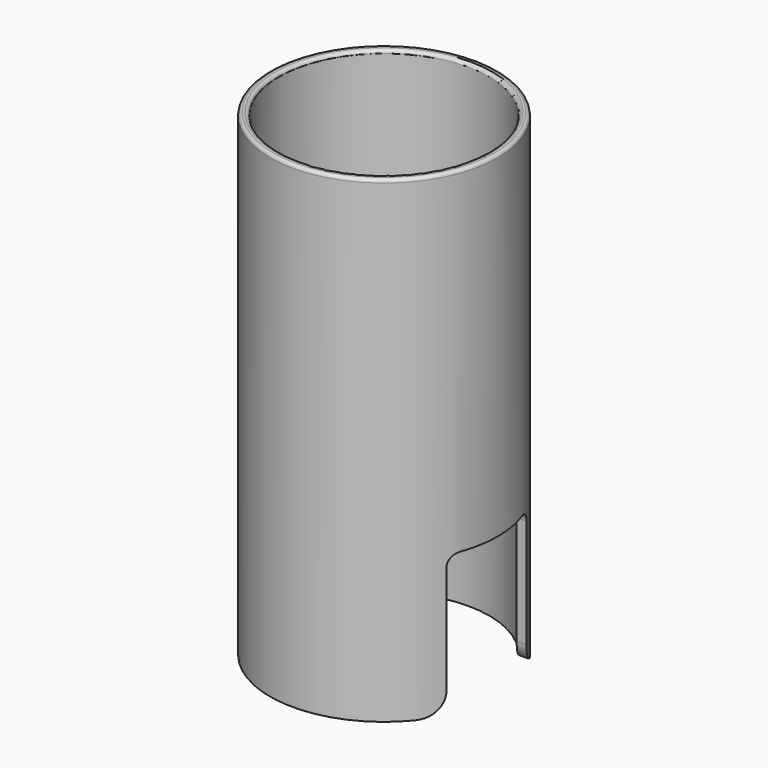
from build123d import *

# Parameters (mm, degrees)
F0_R        = 10.5
F0_R_2      = 9.7
F1_DEPTH    = 44
F3_DEPTH    = 20.75
F4_T1_DEPTH = 10.8988435946
F4_T3_DEPTH = 10.8988435946
F5_R        = 0.3
F6_R        = 1


# Not quite as in the source:
# - a fillet or chamfer that OpenCascade refuses, or shapes differently, is made with other operations: its cross-section is extruded or revolved along the edge and cut away or added


with BuildPart() as f1:
    # F0 (on Top) → F1 (new body)
    with BuildSketch(Plane.XY):
        Circle(F0_R)
        Circle(F0_R_2, mode=Mode.SUBTRACT)
    extrude(amount=F1_DEPTH)

    # F2 (on Right) → F3 (cut, symmetric)
    with BuildSketch(Plane.YZ):
        Polygon((-11.3, 0), (-11.3, -7.5), (11.3, -7.5), (11.3, 0), (4.6, 0), (4.6, 13), (-4.6, 13), (-4.6, 0), align=None)
    extrude(amount=F3_DEPTH, both=True, mode=Mode.SUBTRACT)

    # F4: fillet of radius 2 on 4 edges, made by hand

    # F4_s2 → F4_t1 (cut)
    with BuildSketch(Plane.YZ.offset(-14.4387499172)):
        with BuildLine():
            ThreePointArc((-4.6, 2), (-5.1857864376, 0.5857864376), (-6.6, 0))
            Line((-6.6, 0), (-4.6, 0))
            Line((-4.6, 0), (-4.6, 2))
        make_face()
        with BuildLine():
            ThreePointArc((6.6, 0), (5.1857864376, 0.5857864376), (4.6, 2))
            Line((4.6, 2), (4.6, 0))
            Line((4.6, 0), (6.6, 0))
        make_face()
    extrude(amount=F4_T1_DEPTH, mode=Mode.SUBTRACT)

    # F4_s4 → F4_t3 (cut)
    with BuildSketch(Plane.YZ.offset(3.5399063227)):
        with BuildLine():
            ThreePointArc((-6.6, 0), (-5.1857864376, 0.5857864376), (-4.6, 2))
            Line((-4.6, 2), (-4.6, 0))
            Line((-4.6, 0), (-6.6, 0))
        make_face()
        with BuildLine():
            ThreePointArc((4.6, 2), (5.1857864376, 0.5857864376), (6.6, 0))
            Line((6.6, 0), (4.6, 0))
            Line((4.6, 0), (4.6, 2))
        make_face()
    extrude(amount=F4_T3_DEPTH, mode=Mode.SUBTRACT)

    # F5
    f5_edges = [f1.edges().sort_by_distance(p)[0] for p in [
        (-10.5, 0, 44),
        (-9.7, 0, 44),
    ]]
    fillet(f5_edges, radius=F5_R)

    # F6
    f6_edges = [f1.edges().sort_by_distance(p)[0] for p in [
        (8.989328, -4.6, 13),
        (-8.989328, -4.6, 13),
        (8.989328, 4.6, 13),
        (-8.989328, 4.6, 13),
    ]]
    fillet(f6_edges, radius=F6_R)


solid = f1.part
